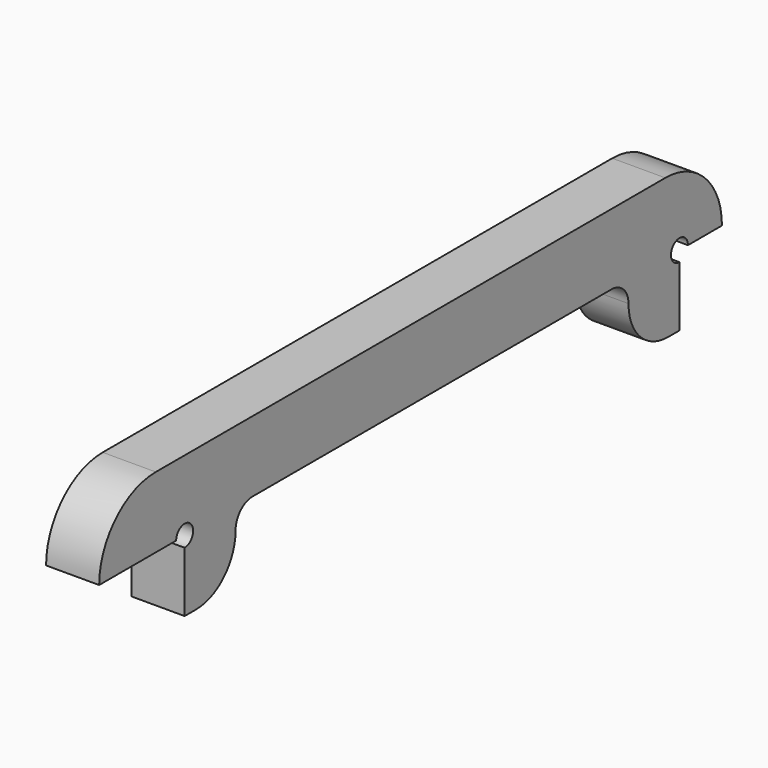
from build123d import *

# Parameters (mm, degrees)
F1_DEPTH = 15


# Not quite as in the source:
# - a feature names something its author has since deleted; it is built from what else it names


with BuildPart() as f1:
    # F0 (on Right) → F1 (new body)
    with BuildSketch(Plane.YZ):
        with BuildLine():
            Line((-15.3621651637, 44.4962902069), (-105.3621651637, 44.4962902069))
            ThreePointArc((-105.3621651637, 44.4962902069), (-119.5043007874, 38.6384258306), (-125.3621651637, 24.4962902069))
            Line((-125.3621651637, 24.4962902069), (-98.1621651637, 24.4962902069))
            ThreePointArc((-98.1621651637, 24.4962902069), (-93.0408448201, 26.6176105505), (-95.1621651637, 21.4962902069))
            Line((-95.1621651637, 21.4962902069), (-95.1621651637, 4.4962902069))
            Line((-95.1621651637, 4.4962902069), (-91.1621651637, 4.4962902069))
            ThreePointArc((-91.1621651637, 4.4962902069), (-81.2626702271, 8.5967952703), (-77.1621651637, 18.4962902069))
            ThreePointArc((-77.1621651637, 18.4962902069), (-75.4048058508, 22.738930894), (-71.1621651637, 24.4962902069))
            Line((-71.1621651637, 24.4962902069), (-15.3621651637, 24.4962902069))
            Line((-15.3621651637, 24.4962902069), (40.4378348363, 24.4962902069))
            Line((40.4378348363, 24.4962902069), (55.6378348363, 24.4962902069))
            ThreePointArc((55.6378348363, 24.4962902069), (59.8804755234, 22.738930894), (61.6378348363, 18.4962902069))
            ThreePointArc((61.6378348363, 18.4962902069), (65.7383398997, 8.5967952703), (75.6378348363, 4.4962902069))
            Line((75.6378348363, 4.4962902069), (79.6378348363, 4.4962902069))
            Line((79.6378348363, 4.4962902069), (79.6378348363, 21.4962902069))
            ThreePointArc((79.6378348363, 21.4962902069), (77.5165144927, 26.6176105505), (82.6378348363, 24.4962902069))
            Line((82.6378348363, 24.4962902069), (94.6378348363, 24.4962902069))
            ThreePointArc((94.6378348363, 24.4962902069), (88.77997046, 38.6384258306), (74.6378348363, 44.4962902069))
            Line((74.6378348363, 44.4962902069), (-15.3621651637, 44.4962902069))
        make_face()
    extrude(amount=F1_DEPTH)


solid = f1.part
